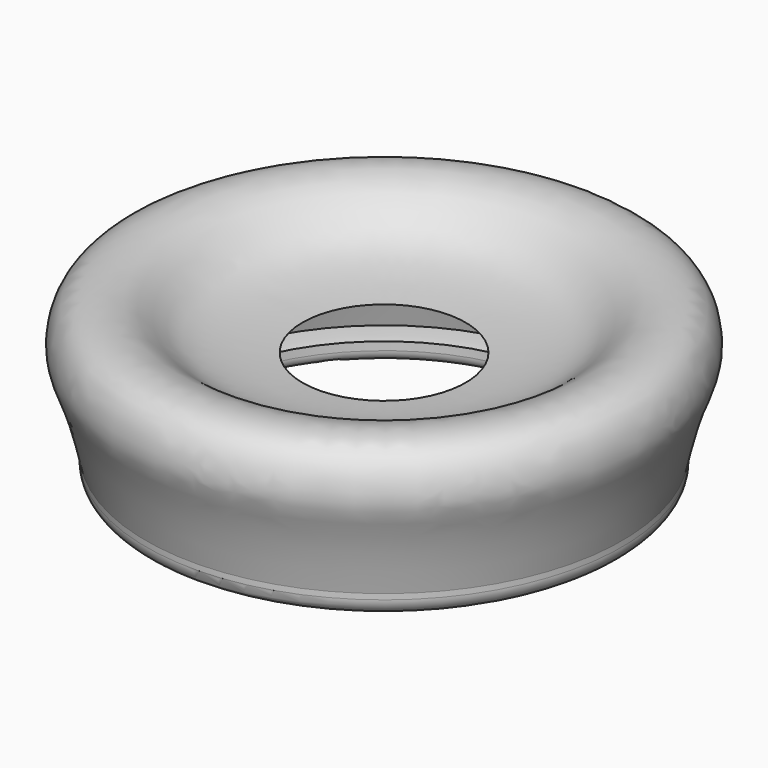
from build123d import *

# Parameters (mm, degrees)
F3_R = 0.5
F4_R = 0.75


with BuildPart() as f1:
    # F0 (on Front) → F1 (revolve)
    with BuildSketch(Plane.XZ):
        with BuildLine():
            add(Edge.make_bspline(
                [(-9.9, 2), (-9.5758501784, 2), (-9.2390440685, 1.9540368163), (-8.9, 1.8756836241)],
                knots=[0, 0, 0, 0, 0.9057827175, 0.9057827175, 0.9057827175, 0.9057827175], degree=3))
            add(Edge.make_bspline(
                [(-9.9, 2), (-9.4425315337, 3.4727421793), (-9.4923738418, 4.5062098982), (-5.7338769398, 5.657842442), (-3.7378328669, 6.0512309775)],
                knots=[0, 0, 0, 0, 0.3609898147, 0.7464263039, 0.7464263039, 0.7464263039, 0.7464263039], degree=3))
            add(Edge.make_bspline(
                [(-3.7378328669, 6.0512309775), (-5.4080331592, 6.1678928498), (-7.540306393, 6.4773144128), (-8.8608693051, 8.3364996593), (-11.6840963626, 8.4712647723), (-12.321294733, 6.1724447902), (-11.5347135554, 4.7688239601), (-11.0895165965, 2.8869020172), (-10.9, 2)],
                knots=[0, 0, 0, 0, 0.2118936526, 0.3670977167, 0.5306355286, 0.6792791718, 0.8175861129, 1, 1, 1, 1], degree=3))
            Line((-10.9, 2), (-10.9, 1))
            Line((-10.9, 1), (-8.9, 1))
            Line((-8.9, 1), (-8.9, 1.8756836241))
        make_face()
    revolve(axis=Axis((0, 0, 3.25), (0, 0, 1)))

    # F3
    f3_edges = [f1.edges().sort_by_distance(p)[0] for p in [
        (8.9, 0, 1),
    ]]
    fillet(f3_edges, radius=F3_R)

    # F4
    f4_edges = [f1.edges().sort_by_distance(p)[0] for p in [
        (10.9, 0, 1),
    ]]
    fillet(f4_edges, radius=F4_R)


solid = f1.part
